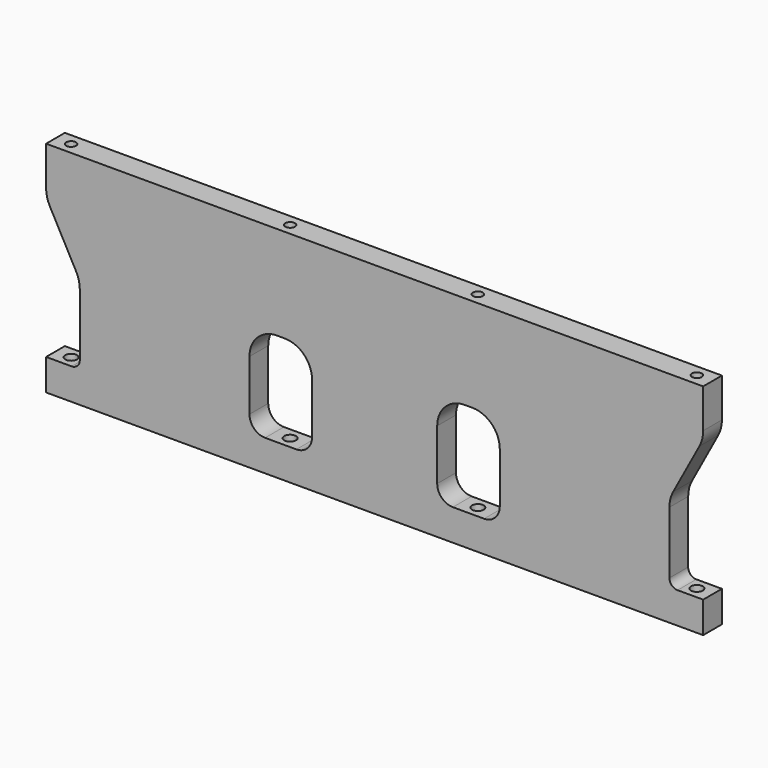
from build123d import *

# Parameters (mm, degrees)
F1_DEPTH = 19.05
F2_R     = 25.4
F3_R     = 4.7879
F4_DEPTH = 33.02
F5_R     = 3.96875
F6_DEPTH = 28.575


# Not quite as in the source:
# - a feature names something its author has since deleted; it is built from what else it names


with BuildPart() as f1:
    # F0 (on Front) → F1 (new body)
    with BuildSketch(Plane.XZ):
        with BuildLine():
            Line((-266.7, -63.5), (-266.7, -88.9))
            Line((-266.7, -88.9), (266.7, -88.9))
            Line((266.7, -88.9), (266.7, -63.5))
            Line((266.7, -63.5), (245.919625, -63.5))
            ThreePointArc((245.919625, -63.5), (241.249891817, -61.565733183), (239.315625, -56.896))
            Line((239.315625, -56.896), (239.315625, 0))
            Line((239.315625, 0), (266.7, 50.8))
            Line((266.7, 50.8), (266.7, 88.9))
            Line((266.7, 88.9), (-266.7, 88.9))
            Line((-266.7, 88.9), (-266.7, 50.8))
            Line((-266.7, 50.8), (-239.315625, 0))
            Line((-239.315625, 0), (-239.315625, -56.896))
            ThreePointArc((-239.315625, -56.896), (-241.249891817, -61.565733183), (-245.919625, -63.5))
            Line((-245.919625, -63.5), (-266.7, -63.5))
        make_face()
        with BuildLine():
            Line((-63.5, -63.5), (-88.9, -63.5))
            ThreePointArc((-88.9, -63.5), (-97.8802561211, -59.7802561211), (-101.6, -50.8))
            Line((-101.6, -50.8), (-101.6, -9.525))
            ThreePointArc((-101.6, -9.525), (-95.0904482119, 6.1904482119), (-79.375, 12.7))
            Line((-79.375, 12.7), (-73.025, 12.7))
            ThreePointArc((-73.025, 12.7), (-57.3095517881, 6.1904482119), (-50.8, -9.525))
            Line((-50.8, -9.525), (-50.8, -50.8))
            ThreePointArc((-50.8, -50.8), (-54.5197438789, -59.7802561211), (-63.5, -63.5))
        make_face(mode=Mode.SUBTRACT)
        with BuildLine():
            ThreePointArc((63.5, -63.5), (54.5197438789, -59.7802561211), (50.8, -50.8))
            Line((50.8, -50.8), (50.8, -9.525))
            ThreePointArc((50.8, -9.525), (57.3095517881, 6.1904482119), (73.025, 12.7))
            Line((73.025, 12.7), (79.375, 12.7))
            ThreePointArc((79.375, 12.7), (95.0904482119, 6.1904482119), (101.6, -9.525))
            Line((101.6, -9.525), (101.6, -50.8))
            ThreePointArc((101.6, -50.8), (97.8802561211, -59.7802561211), (88.9, -63.5))
            Line((88.9, -63.5), (63.5, -63.5))
        make_face(mode=Mode.SUBTRACT)
    extrude(amount=F1_DEPTH)

    # F2
    f2_edges = [f1.edges().sort_by_distance(p)[0] for p in [
        (-266.7, -9.525, 50.8),
        (-239.315625, -9.525, 0),
        (266.7, -9.525, 50.8),
        (239.315625, -9.525, 0),
    ]]
    fillet(f2_edges, radius=F2_R)

    # F3 (on face) → F4 (cut)
    with BuildSketch(Plane(origin=(0, 0, -88.9), x_dir=(1, 0, 0), z_dir=(0, 0, -1))):
        with Locations((-254, 9.525)):
            Circle(F3_R)
        with Locations((-76.2, 9.525)):
            Circle(F3_R)
        with Locations((254, 9.525)):
            Circle(F3_R)
        with Locations((76.2, 9.525)):
            Circle(F3_R)
    extrude(amount=-F4_DEPTH, mode=Mode.SUBTRACT)

    # F5 (on face) → F6 (cut)
    with BuildSketch(Plane.XY.offset(88.9)):
        with Locations((-254, -9.525)):
            Circle(F5_R)
        with Locations((-76.2, -9.525)):
            Circle(F5_R)
        with Locations((76.2, -9.525)):
            Circle(F5_R)
        with Locations((254, -9.525)):
            Circle(F5_R)
    extrude(amount=-F6_DEPTH, mode=Mode.SUBTRACT)


solid = f1.part
